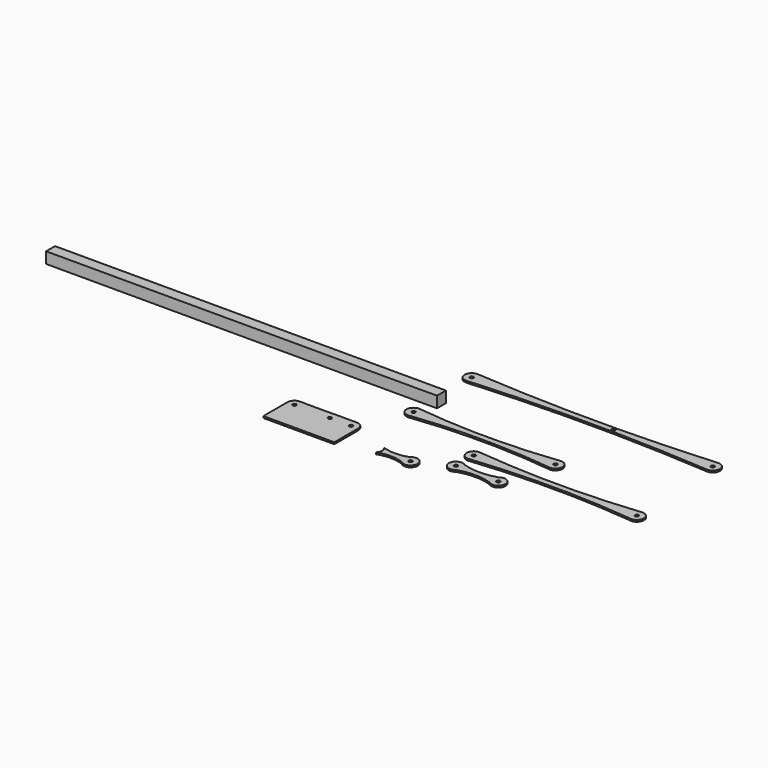
from build123d import *

# Parameters (mm, degrees)
F1_R      = 3.175
F7_DEPTH  = 3.175
F2_R      = 3.175
F8_DEPTH  = 3.175
F9_DEPTH  = 3.175
F6_R      = 3.175
F10_DEPTH = 3.175
F3_R      = 3.175
F11_DEPTH = 3.175
F4_R      = 3.175
F12_DEPTH = 3.175
F0_W      = 700
F0_H      = 20
F13_DEPTH = 20


# Not quite as in the source:
# - a feature names something its author has since deleted; it is built from what else it names


with BuildPart() as f7:
    # F1 (on Top) → F7 (new body)
    with BuildSketch(Plane.XY):
        with BuildLine():
            ThreePointArc((78.1529593822, 12.4298178438), (76.8500505757, 12.5643009555), (75.5472678483, 12.7))
            ThreePointArc((75.5472678483, 12.7), (62.8472678483, 0), (75.5472678483, -12.7))
            ThreePointArc((75.5472678483, -12.7), (76.8500505757, -12.5643009555), (78.1529593822, -12.4298178438))
            ThreePointArc((78.1529593822, -12.4298178438), (85.4058246007, -8.0061762883), (88.2472678483, 0))
            ThreePointArc((88.2472678483, 0), (85.4058246007, 8.0061762883), (78.1529593822, 12.4298178438))
        make_face()
        with Locations((75.5472678483, 0)):
            Circle(F1_R, mode=Mode.SUBTRACT)
        with BuildLine():
            ThreePointArc((365.0415763144, 12.4298178438), (221.5972678483, 5.08), (78.1529593822, 12.4298178438))
            ThreePointArc((78.1529593822, 12.4298178438), (85.4058246007, 8.0061762883), (88.2472678483, 0))
            Line((88.2472678483, 0), (354.9472678483, 0))
            ThreePointArc((354.9472678483, 0), (357.7887110959, 8.0061762883), (365.0415763144, 12.4298178438))
        make_face()
        with BuildLine():
            ThreePointArc((88.2472678483, 0), (85.4058246007, -8.0061762883), (78.1529593822, -12.4298178438))
            ThreePointArc((78.1529593822, -12.4298178438), (221.5972678483, -5.08), (365.0415763144, -12.4298178438))
            ThreePointArc((365.0415763144, -12.4298178438), (357.7887110959, -8.0061762883), (354.9472678483, 0))
            Line((354.9472678483, 0), (88.2472678483, 0))
        make_face()
        with BuildLine():
            ThreePointArc((367.6472678483, 12.7), (366.3444851209, 12.5643009555), (365.0415763144, 12.4298178438))
            ThreePointArc((365.0415763144, 12.4298178438), (357.7887110959, 8.0061762883), (354.9472678483, 0))
            ThreePointArc((354.9472678483, 0), (357.7887110959, -8.0061762883), (365.0415763144, -12.4298178438))
            ThreePointArc((365.0415763144, -12.4298178438), (366.3444851209, -12.5643009555), (367.6472678483, -12.7))
            ThreePointArc((367.6472678483, -12.7), (376.6275239694, -8.9802561211), (380.3472678483, 0))
            ThreePointArc((380.3472678483, 0), (376.6275239694, 8.9802561211), (367.6472678483, 12.7))
        make_face()
        with BuildLine():
            ThreePointArc((370.8222678483, 0), (367.6472678483, -3.175), (364.4722678483, 0))
            ThreePointArc((364.4722678483, 0), (367.6472678483, 3.175), (370.8222678483, 0))
        make_face(mode=Mode.SUBTRACT)
    extrude(amount=F7_DEPTH)


with BuildPart() as f8:
    # F2 (on Top) → F8 (new body)
    with BuildSketch(Plane.XY):
        with BuildLine():
            ThreePointArc((143.5515700519, -30.2544331759), (113.6472678483, -34.8760071528), (83.7429656448, -30.2544331759))
            ThreePointArc((83.7429656448, -30.2544331759), (87.0662817387, -34.6078935608), (88.2472678483, -39.9560071528))
            Line((88.2472678483, -39.9560071528), (139.0472678483, -39.9560071528))
            ThreePointArc((139.0472678483, -39.9560071528), (140.2282539579, -34.6078935608), (143.5515700519, -30.2544331759))
        make_face()
        with BuildLine():
            ThreePointArc((151.7472678483, -27.2560071528), (147.6824543353, -28.8455168838), (143.5515700519, -30.2544331759))
            ThreePointArc((143.5515700519, -30.2544331759), (140.2282539579, -34.6078935608), (139.0472678483, -39.9560071528))
            ThreePointArc((139.0472678483, -39.9560071528), (140.2282539579, -45.3041207448), (143.5515700519, -49.6575811297))
            ThreePointArc((143.5515700519, -49.6575811297), (147.6824543353, -51.0664974218), (151.7472678483, -52.6560071528))
            ThreePointArc((151.7472678483, -52.6560071528), (160.7275239694, -48.9362632739), (164.4472678483, -39.9560071528))
            ThreePointArc((164.4472678483, -39.9560071528), (160.7275239694, -30.9757510317), (151.7472678483, -27.2560071528))
        make_face()
        with BuildLine():
            ThreePointArc((154.9222678483, -39.9560071528), (151.7472678483, -43.1310071528), (148.5722678483, -39.9560071528))
            ThreePointArc((148.5722678483, -39.9560071528), (151.7472678483, -36.7810071528), (154.9222678483, -39.9560071528))
        make_face(mode=Mode.SUBTRACT)
        with BuildLine():
            ThreePointArc((88.2472678483, -39.9560071528), (87.0662817387, -45.3041207448), (83.7429656448, -49.6575811297))
            ThreePointArc((83.7429656448, -49.6575811297), (113.6472678483, -45.0360071528), (143.5515700519, -49.6575811297))
            ThreePointArc((143.5515700519, -49.6575811297), (140.2282539579, -45.3041207448), (139.0472678483, -39.9560071528))
            Line((139.0472678483, -39.9560071528), (88.2472678483, -39.9560071528))
        make_face()
        with BuildLine():
            ThreePointArc((83.7429656448, -49.6575811297), (79.6120813614, -51.0664974218), (75.5472678483, -52.6560071528))
            ThreePointArc((75.5472678483, -52.6560071528), (79.9107532954, -51.8828673747), (83.7429656448, -49.6575811297))
        make_face()
        with BuildLine():
            ThreePointArc((151.7472678483, -52.6560071528), (147.6824543353, -51.0664974218), (143.5515700519, -49.6575811297))
            ThreePointArc((143.5515700519, -49.6575811297), (147.3837824013, -51.8828673747), (151.7472678483, -52.6560071528))
        make_face()
        with BuildLine():
            ThreePointArc((83.7429656448, -30.2544331759), (79.6120813614, -28.8455168838), (75.5472678483, -27.2560071528))
            ThreePointArc((75.5472678483, -27.2560071528), (62.8472678483, -39.9560071528), (75.5472678483, -52.6560071528))
            ThreePointArc((75.5472678483, -52.6560071528), (79.6120813614, -51.0664974218), (83.7429656448, -49.6575811297))
            ThreePointArc((83.7429656448, -49.6575811297), (87.0662817387, -45.3041207448), (88.2472678483, -39.9560071528))
            ThreePointArc((88.2472678483, -39.9560071528), (87.0662817387, -34.6078935608), (83.7429656448, -30.2544331759))
        make_face()
        with Locations((75.5472678483, -39.9560071528)):
            Circle(F2_R, mode=Mode.SUBTRACT)
        with BuildLine():
            ThreePointArc((83.7429656448, -30.2544331759), (79.9107532954, -28.0291469309), (75.5472678483, -27.2560071528))
            ThreePointArc((75.5472678483, -27.2560071528), (79.6120813614, -28.8455168838), (83.7429656448, -30.2544331759))
        make_face()
        with BuildLine():
            ThreePointArc((151.7472678483, -27.2560071528), (147.3837824013, -28.0291469309), (143.5515700519, -30.2544331759))
            ThreePointArc((143.5515700519, -30.2544331759), (147.6824543353, -28.8455168838), (151.7472678483, -27.2560071528))
        make_face()
    extrude(amount=F8_DEPTH)


with BuildPart() as f9:
    # F5 (on Top) → F9 (new body)
    with BuildSketch(Plane.XY):
        with BuildLine():
            ThreePointArc((8.3790727633, -60.0068366925), (-14.2554334044, -63.7697871161), (-36.8899395722, -60.0068366925))
            ThreePointArc((-36.8899395722, -60.0068366925), (-34.2356251717, -64.078873769), (-33.3054334044, -68.8497871161))
            Line((-33.3054334044, -68.8497871161), (4.7945665956, -68.8497871161))
            ThreePointArc((4.7945665956, -68.8497871161), (5.7247583628, -64.078873769), (8.3790727633, -60.0068366925))
        make_face()
        with BuildLine():
            ThreePointArc((-33.3054334044, -68.8497871161), (-34.2356251717, -73.6207004631), (-36.8899395722, -77.6927375396))
            ThreePointArc((-36.8899395722, -77.6927375396), (-14.2554334044, -73.9297871161), (8.3790727633, -77.6927375396))
            ThreePointArc((8.3790727633, -77.6927375396), (5.7247583628, -73.6207004631), (4.7945665956, -68.8497871161))
            Line((4.7945665956, -68.8497871161), (-33.3054334044, -68.8497871161))
        make_face()
        with BuildLine():
            ThreePointArc((17.4945665956, -56.1497871161), (13.0051211687, -58.2397310906), (8.3790727633, -60.0068366925))
            ThreePointArc((8.3790727633, -60.0068366925), (5.7247583628, -64.078873769), (4.7945665956, -68.8497871161))
            ThreePointArc((4.7945665956, -68.8497871161), (5.7247583628, -73.6207004631), (8.3790727633, -77.6927375396))
            ThreePointArc((8.3790727633, -77.6927375396), (13.0051211687, -79.4598431415), (17.4945665956, -81.5497871161))
            ThreePointArc((17.4945665956, -81.5497871161), (26.4748227166, -77.8300432371), (30.1945665956, -68.8497871161))
            ThreePointArc((30.1945665956, -68.8497871161), (26.4748227166, -59.869530995), (17.4945665956, -56.1497871161))
        make_face()
        with BuildLine():
            ThreePointArc((20.6695665956, -68.8497871161), (17.4945665956, -72.0247871161), (14.3195665956, -68.8497871161))
            ThreePointArc((14.3195665956, -68.8497871161), (17.4945665956, -65.6747871161), (20.6695665956, -68.8497871161))
        make_face(mode=Mode.SUBTRACT)
        with BuildLine():
            ThreePointArc((17.4945665956, -56.1497871161), (12.5456005611, -57.1537307213), (8.3790727633, -60.0068366925))
            ThreePointArc((8.3790727633, -60.0068366925), (13.0051211687, -58.2397310906), (17.4945665956, -56.1497871161))
        make_face()
        with BuildLine():
            ThreePointArc((17.4945665956, -81.5497871161), (13.0051211687, -79.4598431415), (8.3790727633, -77.6927375396))
            ThreePointArc((8.3790727633, -77.6927375396), (12.5456005611, -80.5458435108), (17.4945665956, -81.5497871161))
        make_face()
    extrude(amount=F9_DEPTH)


with BuildPart() as f10:
    # F6 (on Top) → F10 (new body)
    with BuildSketch(Plane.XY):
        with BuildLine():
            ThreePointArc((-215.3885840548, -24.2675056169), (-215.6442924486, -24.2623758889), (-215.9, -24.2572043419))
            ThreePointArc((-215.9, -24.2572043419), (-224.8802561211, -27.9769482208), (-228.6, -36.9572043419))
            ThreePointArc((-228.6, -36.9572043419), (-215.9, -49.6572043419), (-203.2, -36.9572043419))
            ThreePointArc((-203.2, -36.9572043419), (-206.740715571, -28.1596189488), (-215.3885840548, -24.2675056169))
        make_face()
        with Locations((-215.9, -36.9572043419)):
            Circle(F6_R, mode=Mode.SUBTRACT)
        with BuildLine():
            ThreePointArc((-203.2, -36.9572043419), (-215.9, -49.6572043419), (-228.6, -36.9572043419))
            Line((-228.6, -36.9572043419), (-228.6, -90.6351879239))
            Line((-228.6, -90.6351879239), (-101.6, -90.6351879239))
            Line((-101.6, -90.6351879239), (-101.6, -36.9572043419))
            ThreePointArc((-101.6, -36.9572043419), (-123.2802561211, -45.937460463), (-114.3, -24.2572043419))
            Line((-114.3, -24.2572043419), (-152.4, -24.2572043419))
            ThreePointArc((-152.4, -24.2572043419), (-143.4197438789, -27.9769482208), (-139.7, -36.9572043419))
            ThreePointArc((-139.7, -36.9572043419), (-161.197585393, -46.1164887709), (-152.9114159452, -24.2675056169))
            ThreePointArc((-152.9114159452, -24.2675056169), (-184.15, -24.579533058), (-215.3885840548, -24.2675056169))
            ThreePointArc((-215.3885840548, -24.2675056169), (-206.740715571, -28.1596189488), (-203.2, -36.9572043419))
        make_face()
        with BuildLine():
            ThreePointArc((-152.4, -24.2572043419), (-152.6557075514, -24.2623758889), (-152.9114159452, -24.2675056169))
            ThreePointArc((-152.9114159452, -24.2675056169), (-161.197585393, -46.1164887709), (-139.7, -36.9572043419))
            ThreePointArc((-139.7, -36.9572043419), (-143.4197438789, -27.9769482208), (-152.4, -24.2572043419))
        make_face()
        with Locations((-152.4, -36.9572043419)):
            Circle(F6_R, mode=Mode.SUBTRACT)
        with BuildLine():
            ThreePointArc((-114.3, -24.2572043419), (-123.2802561211, -45.937460463), (-101.6, -36.9572043419))
            ThreePointArc((-101.6, -36.9572043419), (-105.3197438789, -27.9769482208), (-114.3, -24.2572043419))
        make_face()
        with Locations((-114.3, -36.9572043419)):
            Circle(F6_R, mode=Mode.SUBTRACT)
    extrude(amount=F10_DEPTH)


with BuildPart() as f11:
    # F3 (on Top) → F11 (new body)
    with BuildSketch(Plane.XY):
        with BuildLine():
            ThreePointArc((-69.4611344861, 62.6005697173), (-70.9514619098, 62.7768515998), (-72.441538775, 62.9552390099))
            ThreePointArc((-72.441538775, 62.9552390099), (-85.141538775, 50.2552390099), (-72.441538775, 37.5552390099))
            ThreePointArc((-72.441538775, 37.5552390099), (-70.9514619098, 37.7336264199), (-69.4611344861, 37.9099083025))
            ThreePointArc((-69.4611344861, 37.9099083025), (-62.4630335144, 42.3990673744), (-59.741538775, 50.2552390099))
            ThreePointArc((-59.741538775, 50.2552390099), (-62.4630335144, 58.1114106453), (-69.4611344861, 62.6005697173))
        make_face()
        with Locations((-72.441538775, 50.2552390099)):
            Circle(F3_R, mode=Mode.SUBTRACT)
        with BuildLine():
            ThreePointArc((178.5780569362, 62.6005697173), (54.558461225, 55.3352390099), (-69.4611344861, 62.6005697173))
            ThreePointArc((-69.4611344861, 62.6005697173), (-62.4630335144, 58.1114106453), (-59.741538775, 50.2552390099))
            Line((-59.741538775, 50.2552390099), (168.858461225, 50.2552390099))
            ThreePointArc((168.858461225, 50.2552390099), (171.5799559645, 58.1114106453), (178.5780569362, 62.6005697173))
        make_face()
        with BuildLine():
            ThreePointArc((-59.741538775, 50.2552390099), (-62.4630335144, 42.3990673744), (-69.4611344861, 37.9099083025))
            ThreePointArc((-69.4611344861, 37.9099083025), (54.558461225, 45.1752390099), (178.5780569362, 37.9099083025))
            ThreePointArc((178.5780569362, 37.9099083025), (171.5799559645, 42.3990673744), (168.858461225, 50.2552390099))
            Line((168.858461225, 50.2552390099), (-59.741538775, 50.2552390099))
        make_face()
        with BuildLine():
            ThreePointArc((181.558461225, 62.9552390099), (180.0683843599, 62.7768515998), (178.5780569362, 62.6005697173))
            ThreePointArc((178.5780569362, 62.6005697173), (171.5799559645, 58.1114106453), (168.858461225, 50.2552390099))
            ThreePointArc((168.858461225, 50.2552390099), (171.5799559645, 42.3990673744), (178.5780569362, 37.9099083025))
            ThreePointArc((178.5780569362, 37.9099083025), (180.0683843599, 37.7336264199), (181.558461225, 37.5552390099))
            ThreePointArc((181.558461225, 37.5552390099), (190.5387173461, 41.2749828888), (194.258461225, 50.2552390099))
            ThreePointArc((194.258461225, 50.2552390099), (190.5387173461, 59.2354951309), (181.558461225, 62.9552390099))
        make_face()
        with BuildLine():
            ThreePointArc((184.733461225, 50.2552390099), (181.558461225, 47.0802390099), (178.383461225, 50.2552390099))
            ThreePointArc((178.383461225, 50.2552390099), (181.558461225, 53.4302390099), (184.733461225, 50.2552390099))
        make_face(mode=Mode.SUBTRACT)
    extrude(amount=F11_DEPTH)


with BuildPart() as f12:
    # F4 (on Top) → F12 (new body)
    with BuildSketch(Plane.XY):
        with BuildLine():
            ThreePointArc((-72.6650020829, 195.5879780869), (-73.5544773878, 195.6504524814), (-74.4439344645, 195.7131858587))
            ThreePointArc((-74.4439344645, 195.7131858587), (-87.1439344645, 183.0131858587), (-74.4439344645, 170.3131858587))
            ThreePointArc((-74.4439344645, 170.3131858587), (-73.5544773878, 170.3759192361), (-72.6650020829, 170.4383936305))
            ThreePointArc((-72.6650020829, 170.4383936305), (-64.8553359943, 174.6855944076), (-61.7439344645, 183.0131858587))
            ThreePointArc((-61.7439344645, 183.0131858587), (-64.8553359943, 191.3407773099), (-72.6650020829, 195.5879780869))
        make_face()
        with Locations((-74.4439344645, 183.0131858587)):
            Circle(F4_R, mode=Mode.SUBTRACT)
        with BuildLine():
            ThreePointArc((355.577133154, 195.5879780869), (141.4560655355, 188.0931858587), (-72.6650020829, 195.5879780869))
            ThreePointArc((-72.6650020829, 195.5879780869), (-64.8553359943, 191.3407773099), (-61.7439344645, 183.0131858587))
            Line((-61.7439344645, 183.0131858587), (176.3810655355, 183.0131858587))
            ThreePointArc((176.3810655355, 183.0131858587), (179.5560655355, 186.1881858587), (182.7310655355, 183.0131858587))
            Line((182.7310655355, 183.0131858587), (344.6560655355, 183.0131858587))
            ThreePointArc((344.6560655355, 183.0131858587), (347.7674670654, 191.3407773099), (355.577133154, 195.5879780869))
        make_face()
        with BuildLine():
            ThreePointArc((-61.7439344645, 183.0131858587), (-64.8553359943, 174.6855944076), (-72.6650020829, 170.4383936305))
            ThreePointArc((-72.6650020829, 170.4383936305), (141.4560655356, 177.9331858587), (355.5771331541, 170.4383936305))
            ThreePointArc((355.5771331541, 170.4383936305), (347.7674670654, 174.6855944076), (344.6560655355, 183.0131858587))
            Line((344.6560655355, 183.0131858587), (182.7310655355, 183.0131858587))
            ThreePointArc((182.7310655355, 183.0131858587), (179.5560655355, 179.8381858587), (176.3810655355, 183.0131858587))
            Line((176.3810655355, 183.0131858587), (-61.7439344645, 183.0131858587))
        make_face()
        with BuildLine():
            ThreePointArc((357.3560655355, 195.7131858587), (356.4666084589, 195.6504524814), (355.577133154, 195.5879780869))
            ThreePointArc((355.577133154, 195.5879780869), (347.7674670654, 191.3407773099), (344.6560655355, 183.0131858587))
            ThreePointArc((344.6560655355, 183.0131858587), (347.7674670654, 174.6855944076), (355.5771331541, 170.4383936305))
            ThreePointArc((355.5771331541, 170.4383936305), (356.4666084589, 170.3759192361), (357.3560655355, 170.3131858587))
            ThreePointArc((357.3560655355, 170.3131858587), (366.3363216566, 174.0329297377), (370.0560655355, 183.0131858587))
            ThreePointArc((370.0560655355, 183.0131858587), (366.3363216566, 191.9934419798), (357.3560655355, 195.7131858587))
        make_face()
        with BuildLine():
            ThreePointArc((360.5310655355, 183.0131858587), (357.3560655355, 179.8381858587), (354.1810655355, 183.0131858587))
            ThreePointArc((354.1810655355, 183.0131858587), (357.3560655355, 186.1881858587), (360.5310655355, 183.0131858587))
        make_face(mode=Mode.SUBTRACT)
    extrude(amount=F12_DEPTH)


with BuildPart() as f13:
    # F0 (on Top) → F13 (new body)
    with BuildSketch(Plane.XY):
        with Locations((-407.3969234348, 93.9524527639)):
            Rectangle(F0_W, F0_H)
    extrude(amount=F13_DEPTH)


solid = Compound([f7.part, f8.part, f9.part, f10.part, f11.part, f12.part, f13.part])
